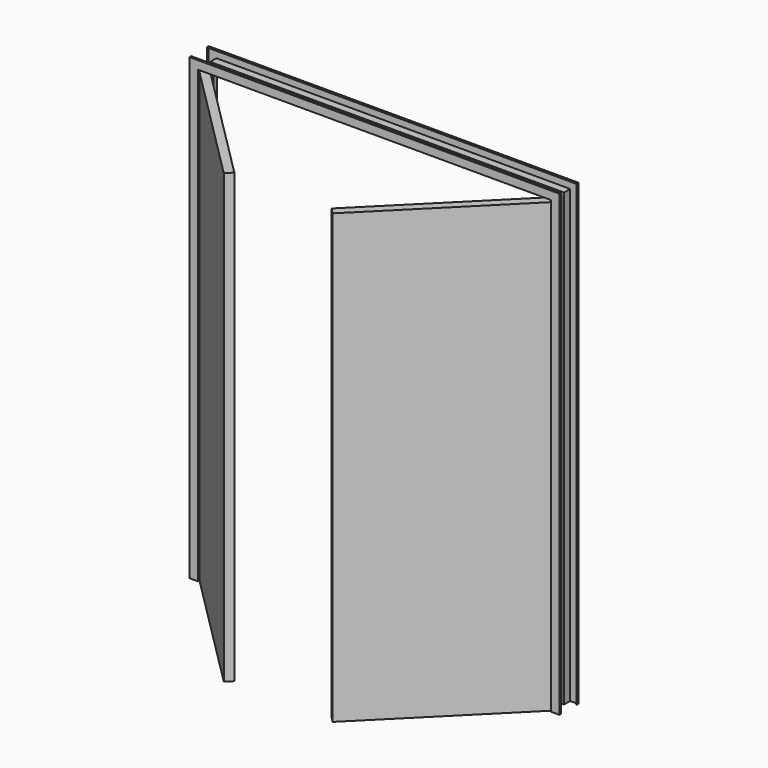
from build123d import *

# Parameters (mm, degrees)
F5_DEPTH = 1370.0125


# Not quite as in the source:
# - a variable given as a bare number and used for a length is read in inches; the dataset says mm whatever the document's units were


with BuildPart() as f3:
    # F3: sweep along a path in F1
    with BuildLine(Plane.XZ) as f3_path:
        Line((-1066.8, -1371.6), (-1066.8, 1371.6))
        Line((-1066.8, 1371.6), (1066.8, 1371.6))
        Line((1066.8, 1371.6), (1066.8, -1371.6))
    # F2 (on Top) → F3 (sweep)
    with BuildSketch(Plane.XY):
        Polygon((-1082.675, 23.368), (-1066.8, 23.368), (-1066.8, -23.368), (-1082.675, -23.368), (-1082.675, -70.993), (-1129.411, -70.993), (-1129.411, -60.325), (-1131.443, -60.325), (-1131.443, -73.025), (-1080.643, -73.025), (-1080.643, -25.4), (-1064.768, -25.4), (-1064.768, 25.4), (-1080.643, 25.4), (-1080.643, 73.025), (-1131.443, 73.025), (-1131.443, 60.325), (-1129.411, 60.325), (-1129.411, 70.993), (-1082.675, 70.993), align=None)
    sweep(path=f3_path.line, transition=Transition.RIGHT)

    # F4 (on Top) → F5 (join, symmetric)
    with BuildSketch(Plane.XY):
        Polygon((-297.1398050959, -773.3301995265), (-1051.4813192657, -18.9886853567), (-1087.40234375, -54.909709841), (-333.0608295802, -809.2512240108), align=None)
    extrude(amount=F5_DEPTH, both=True)

    # F6: F3 across plane


with BuildPart() as f3_1:
    add(f3.part)
    add(f3.part.mirror(Plane.YZ))


solid = f3_1.part
